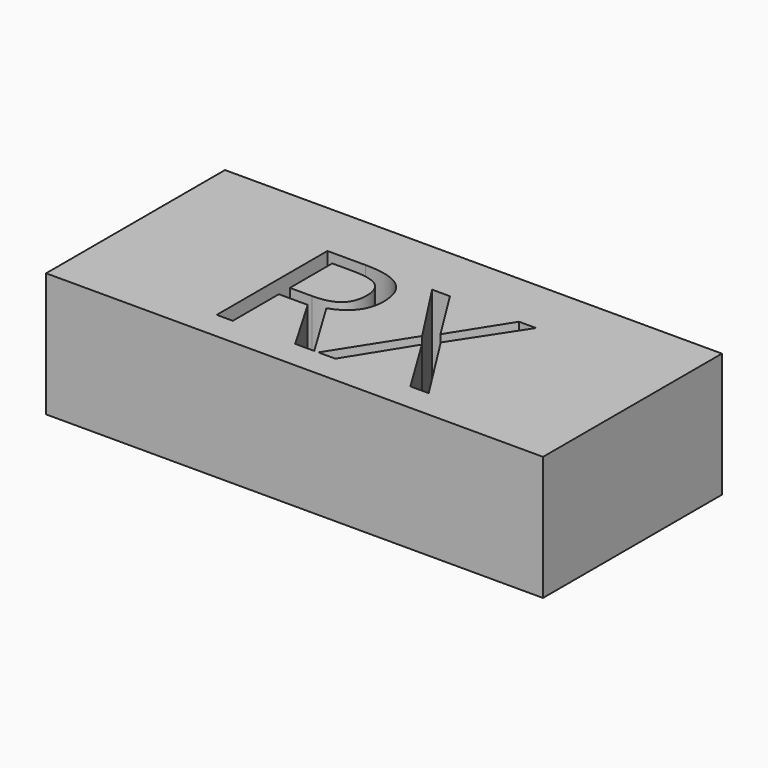
from build123d import *

# Parameters (mm, degrees)
F0_W         = 60
F0_H         = 27
F1_DEPTH     = 15
F2_TEXT_SIZE = 23.4071727997
F3_DEPTH     = 25.4


# Not quite as in the source:
# - Text() gives the source's letters only with a copy of the font that has no kerning and outlines rounded to 1/6400 em; it was checked with that copy


with BuildPart() as f1:
    # F0 (on Top) → F1 (new body)
    with BuildSketch(Plane.XY):
        Rectangle(F0_W, F0_H)
    extrude(amount=F1_DEPTH)

    # F2 (on face) → F3 (cut)
    with BuildSketch(Plane.XY.offset(15)):
        with Locations((-14.4317345694, -10.0794779205)):
            Text('RX', F2_TEXT_SIZE, font='Open Sans', text_align=(TextAlign.LEFT, TextAlign.BOTTOM))
    extrude(amount=-F3_DEPTH, mode=Mode.SUBTRACT)


solid = f1.part
